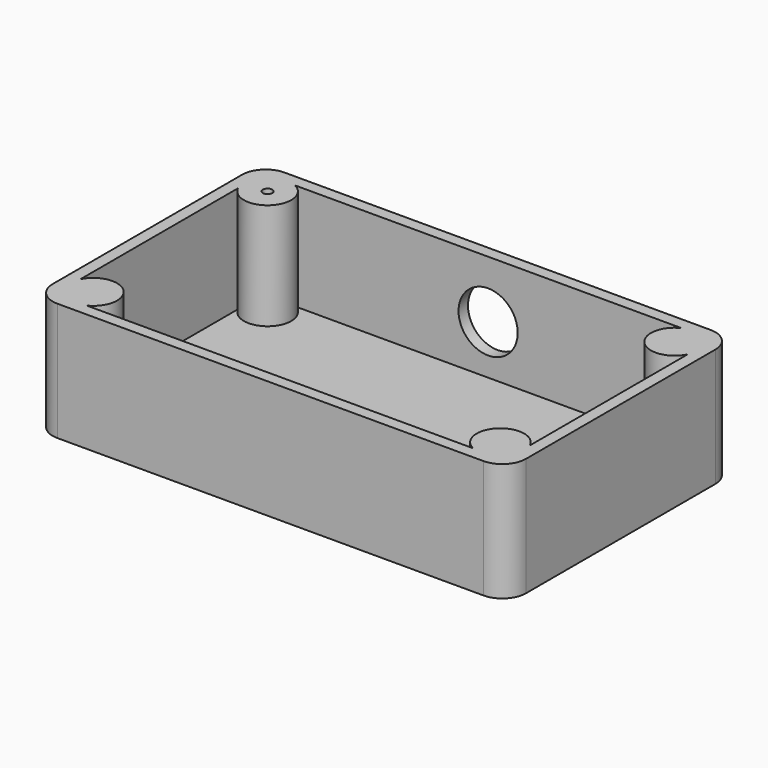
from build123d import *

# Parameters (mm, degrees)
F0_W           = 100
F0_H           = 60
F1_DEPTH       = 25
F2_T           = -2.5
F3_R           = 5
F4_R           = 5
F5_R           = 3.5
F6_DEPTH       = 25
F7_R           = 1.24999
F8_R           = 5
F8_R_2         = 1
F9_DEPTH       = 25
F10_DEPTH      = 1
F10_DEPTH_BACK = 1
F11_R          = 5
F12_DEPTH      = 25
F13_R          = 5
F14_DEPTH      = 25
F15_R          = 5
F16_DEPTH      = 25
F17_R          = 6.25
F18_DEPTH      = 10


# Not quite as in the source:
# - a fillet or chamfer is up to 0.001 mm smaller than in the source, because OpenCascade refuses the exact size


with BuildPart() as f1:
    # F0 (on Top) → F1 (new body)
    with BuildSketch(Plane.XY):
        with Locations((23.0550479144, 14.1446392238)):
            Rectangle(F0_W, F0_H)
    extrude(amount=F1_DEPTH)

    # F2
    f2_openings = [f1.faces().sort_by_distance(p)[0] for p in [
        (23.055048, 14.144639, 25),
    ]]
    offset(amount=F2_T, openings=f2_openings)

    # F3
    f3_edges = [f1.edges().sort_by_distance(p)[0] for p in [
        (-26.944952, 44.144639, 12.5),
        (-26.944952, -15.855361, 12.5),
        (73.055048, -15.855361, 12.5),
        (73.055048, 44.144639, 12.5),
    ]]
    fillet(f3_edges, radius=F3_R)

    # F4
    f4_edges = [f1.edges().sort_by_distance(p)[0] for p in [
        (70.555048, -13.355361, 13.75),
        (-24.444952, 41.644639, 13.75),
        (-24.444952, -13.355361, 13.75),
        (70.555048, 41.644639, 13.75),
    ]]
    fillet(f4_edges, radius=F4_R)

    # F5 (on face) → F6 (cut)
    with BuildSketch(Plane.XY.offset(2.5)):
        with Locations((26.5453665042, 10.6446392238)):
            Circle(F5_R)
    extrude(amount=-F6_DEPTH, mode=Mode.SUBTRACT)

    # F7 (radius 1.25 in the source; OpenCascade refuses exactly that, so slightly less here)
    f7_edges = [f1.edges().sort_by_distance(p)[0] for p in [
        (23.045367, 10.644639, 0),
        (23.045367, 10.644639, 2.5),
    ]]
    fillet(f7_edges, radius=F7_R)

    # F8 (on face) → F9 (join)
    with BuildSketch(Plane.XY):
        with Locations((-19.9449520856, 37.1446392238)):
            Circle(F8_R)
        with Locations((-19.9449520856, 37.1446392238)):
            Circle(F8_R_2, mode=Mode.SUBTRACT)
    extrude(amount=F9_DEPTH)

    # F10 (cut, two sides): a face of the model
    f10_faces = [f1.faces().sort_by_distance(p)[0] for p in [
        (-19.9449520856, 37.1446392238, 2.5),
    ]]
    extrude(f10_faces, amount=-F10_DEPTH, mode=Mode.SUBTRACT)
    extrude(f10_faces, amount=F10_DEPTH_BACK, mode=Mode.SUBTRACT)

    # F11 (on face) → F12 (join)
    with BuildSketch(Plane.XY):
        with Locations((66.0550479144, 37.1446392238)):
            Circle(F11_R)
    extrude(amount=F12_DEPTH)

    # F13 (on face) → F14 (join)
    with BuildSketch(Plane.XY):
        with Locations((-19.9449520856, -8.8553607762)):
            Circle(F13_R)
    extrude(amount=F14_DEPTH)

    # F15 (on face) → F16 (join)
    with BuildSketch(Plane.XY):
        with Locations((66.0550479144, -8.8553607762)):
            Circle(F15_R)
    extrude(amount=F16_DEPTH)

    # F17 (on face) → F18 (cut)
    with BuildSketch(Plane(origin=(0, 44.1446392238, 0), x_dir=(-1, 0, 0), z_dir=(0, 1, 0))):
        with Locations((-23.0550479144, 12.8674265233)):
            Circle(F17_R)
    extrude(amount=-F18_DEPTH, mode=Mode.SUBTRACT)


solid = f1.part
